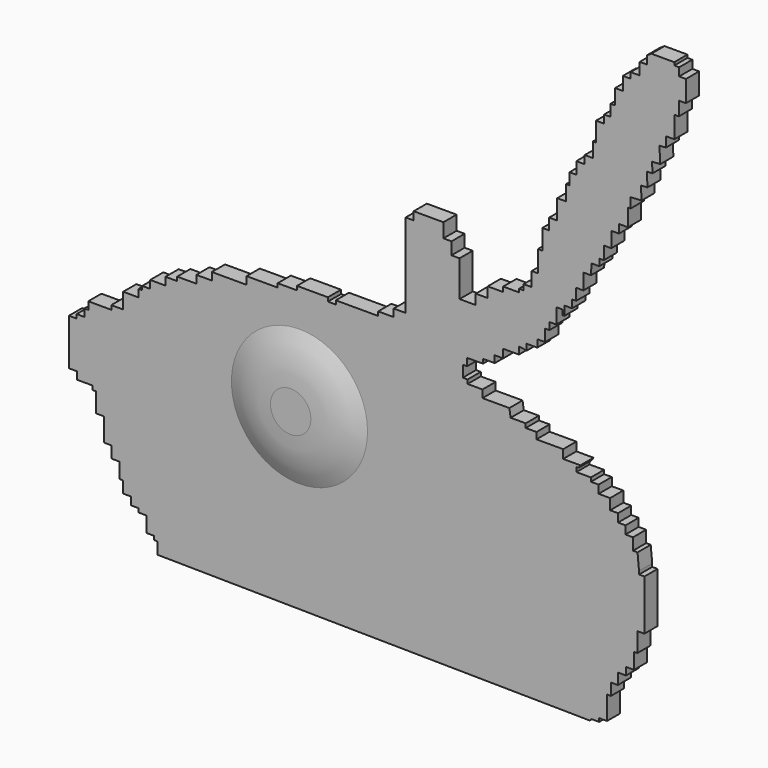
from build123d import *

# Parameters (mm, degrees)
F1_DEPTH = 0.762
F2_R     = 3.1487377101
F3_DEPTH = 0.508


# Not quite as in the source:
# - a fillet or chamfer that OpenCascade refuses, or shapes differently, is made with other operations: its cross-section is extruded or revolved along the edge and cut away or added


with BuildPart() as f1:
    # F0 (on Front) → F1 (new body)
    with BuildSketch(Plane.XZ):
        Polygon((-10.7027310878, 16.9802121818), (-10.7027310878, 16.4352189749), (9.2740571126, 16.1886904389), (9.361166507, 16.2728279829), (9.7121512517, 16.2728279829), (9.7121512517, 16.4274536073), (10.076017119, 16.4274536073), (10.076017119, 17.509419471), (10.2598499507, 17.509419471), (10.2598499507, 18.0550143123), (10.5776172131, 18.0550143123), (10.5776172131, 18.5661129653), (10.9531022608, 18.5661129653), (10.9531022608, 18.9169067889), (11.3242575899, 18.9169067889), (11.3242575899, 19.6492467076), (11.4805521443, 19.6492467076), (11.4805521443, 20.5453597009), (11.8060437962, 20.5453597009), (11.8060437962, 22.8735357523), (11.5571394563, 22.8735357523), (11.5571394563, 23.019047454), (11.4864483476, 23.7509682775), (11.2769883126, 23.7509682775), (11.2769883126, 24.2973826826), (10.9309256077, 24.2973826826), (10.9309256077, 24.6707666665), (10.5848629028, 24.6707666665), (10.5848629028, 25.0532571226), (10.2192526683, 25.0532571226), (10.2192526683, 25.5498923361), (9.6870232373, 25.5498923361), (9.6870232373, 25.9251333773), (9.330926463, 25.9251333773), (9.330926463, 26.1014979333), (8.6600910872, 26.1014979333), (8.6600910872, 26.3056345284), (8.7596448138, 26.3056345284), (8.8438820094, 26.4358203858), (8.0474531278, 26.4358203858), (8.0474531278, 26.8340352923), (6.8145194091, 26.8340352923), (6.8145194091, 27.1326974034), (6.3167512417, 27.1326974034), (6.3167512417, 27.3241456598), (5.6198756211, 27.3241456598), (5.5586118251, 27.699386701), (4.3180198409, 27.699386701), (4.3180198409, 28.0516538769), (3.6288024858, 28.0516538769), (3.6288024858, 28.2354447991), (3.4067214001, 28.2354447991), (3.4067214001, 28.7638437003), (3.6058286205, 28.7638437003), (3.6058286205, 29.108453542), (4.3409941718, 29.108453542), (4.3409941718, 29.3075609952), (4.8847105354, 29.3075609952), (4.8847105354, 29.6291969717), (5.2762227133, 29.6291969717), (5.2762227133, 30.0197526813), (6.0027744621, 30.0197526813), (6.0027744621, 30.3567033261), (6.3626994379, 30.2954409271), (6.3626994379, 30.5787846446), (6.8528093398, 30.5787846446), (6.8528093398, 30.9233944863), (7.2127343155, 30.9233944863), (7.2127343155, 31.4747691154), (7.4139898643, 31.4747691154), (7.4139898643, 31.8043418229), (7.7288472094, 31.8043418229), (7.7288472094, 32.5135849416), (8.0249523744, 32.5135849416), (8.0249523744, 32.2783663869), (8.1042656675, 32.2783663869), (8.1042656675, 32.7028520405), (8.4611764178, 32.7028520405), (8.4611764178, 33.0685973167), (8.6515294388, 33.0685973167), (8.6515294388, 33.5998237133), (8.9846476912, 33.5998237133), (8.9846476912, 34.3319140375), (9.3336272985, 34.3319140375), (9.3600647524, 34.8261408508), (9.7196195275, 34.8261408508), (9.7196195275, 35.1380035281), (9.9258357659, 35.1380035281), (9.9258357659, 35.7379503548), (10.2721722797, 35.7379503548), (10.2721722797, 36.4488959312), (10.6290839612, 36.4488959312), (10.6290839612, 36.8426926434), (11.0468016937, 36.8426926434), (11.0468016937, 37.5430695713), (11.0468016937, 37.6461409032), (11.1684938893, 37.6461409032), (11.1684938893, 38.1089963577), (11.6737550625, 38.1342493479), (11.6433482944, 38.742627176), (11.9479903872, 38.75785321), (11.9162704796, 39.3925043009), (12.1807143848, 39.4057212265), (12.1571606054, 39.8769846334), (12.5368040454, 39.8959592401), (12.4995354563, 40.6416282058), (12.7986464649, 40.6565777957), (12.7986464649, 41.1200486124), (13.1874894723, 41.1200486124), (13.1874894723, 42.1217381954), (13.3968675509, 42.1217381954), (13.3968675509, 42.7646152675), (13.7258889154, 42.7646152675), (13.7258889154, 43.7513552606), (13.4118227288, 43.7513552606), (13.4118227288, 44.1251210868), (13.1874894723, 44.1251210868), (13.1874894723, 44.2596748471), (12.1256476268, 44.2596748471), (11.9162704796, 44.1251210868), (11.9162704796, 43.7513552606), (11.5872481838, 43.7513552606), (11.5872481838, 43.1981831789), (11.1684938893, 43.1981831789), (11.1684938893, 42.929071933), (10.8095612377, 42.929071933), (10.8095612377, 42.3160977662), (10.4506285861, 42.3160977662), (10.4506285861, 41.6134186089), (10.2412505075, 41.6134186089), (10.2412505075, 41.0751961172), (9.9421404302, 41.0751961172), (9.9421404302, 40.7014340162), (9.567049332, 40.7014340162), (9.567049332, 39.8043952882), (9.4175431877, 39.8043952882), (9.4175431877, 39.1316190362), (9.0437782928, 39.1316190362), (9.0437782928, 38.75785321), (8.6550619453, 38.75785321), (8.6550619453, 38.2046811283), (8.3410982043, 38.2046811283), (8.3410982043, 37.6664586365), (8.1766415387, 37.6664586365), (8.1766415387, 36.9637794793), (7.7729751356, 36.9637794793), (7.7729751356, 36.0517911613), (7.399209775, 36.0517911613), (7.399209775, 35.5285182595), (7.0852469653, 35.5285182595), (7.0852469653, 34.6015803516), (6.8759382702, 34.6015803516), (6.8759382702, 33.6148403585), (6.5918765031, 33.6148403585), (6.5918765031, 32.9570136964), (6.2181116082, 32.9570136964), (6.2181116082, 32.7028520405), (6.0088024475, 32.7028520405), (6.0088024475, 32.553344965), (5.2762227133, 32.553344965), (5.2762227133, 32.3290862143), (4.5585935004, 32.3290862143), (4.5585935004, 31.8506658077), (4.0054204874, 31.8506658077), (4.0054204874, 31.3871987164), (3.2578899991, 31.3871987164), (3.2578899991, 33.0467149615), (2.8841246385, 33.0467149615), (2.8841246385, 33.6148403585), (2.5103592779, 33.6148403585), (2.5103592779, 34.2726670206), (1.1349029373, 34.2726670206), (1.1349029373, 33.8989011943), (0.7648753817, 33.8989011943), (0.7648753817, 30.0117395818), (0.2128840133, 30.0117395818), (0.2128840133, 29.662868008), (-0.5045263097, 29.662868008), (-0.5045263097, 29.4756293297), (-2.4671009742, 29.4756293297), (-2.4671009742, 29.3034724891), (-2.8314732481, 29.3034724891), (-2.8314732481, 29.4800959527), (-4.260267131, 29.4800959527), (-4.260267131, 29.2979851365), (-5.1528010517, 29.2979851365), (-5.1528010517, 29.1180480272), (-6.5885153599, 29.1180480272), (-6.5885153599, 28.7643931806), (-8.1972610205, 28.7643931806), (-8.1972610205, 28.415735811), (-8.9150499552, 28.415735811), (-8.9150499552, 28.0552376062), (-9.7993966192, 28.0552376062), (-9.7993966192, 27.8717204928), (-10.3413742036, 27.8717204928), (-10.3413742036, 27.5138057768), (-11.0485879704, 27.5138057768), (-11.0485879704, 27.1503776312), (-11.4187179133, 27.1503776312), (-11.4187179133, 26.9733015448), (-11.5851024166, 26.9733015448), (-11.5851024166, 26.627080515), (-12.2981043532, 26.627080515), (-12.2981043532, 25.904243812), (-12.8476871178, 25.904243812), (-12.8476871178, 25.7139522582), (-13.9118125662, 25.7139522582), (-13.9118125662, 25.3637637943), (-14.0915913507, 25.3637637943), (-14.0915913507, 25.0175409019), (-14.4485030323, 25.0175409019), (-14.4485030323, 24.8338580132), (-14.8080587387, 24.8338580132), (-14.8080587387, 22.6944163442), (-14.4432177767, 22.6944163442), (-14.4432177767, 22.3495159298), (-13.7267503887, 22.3495159298), (-13.7267503887, 22.1658330411), (-13.5496165603, 22.1658330411), (-13.5496165603, 21.265918389), (-13.1914103404, 21.265918389), (-13.1914103404, 20.1955363154), (-12.8319738433, 20.1955363154), (-12.8319738433, 19.6577031165), (-12.4698942527, 19.6577031165), (-12.4698942527, 18.9454331994), (-12.2981043532, 18.9454331994), (-12.2981043532, 18.4089224786), (-11.9370780885, 18.4089224786), (-11.9370780885, 18.0474910885), (-11.5851024166, 18.0474910885), (-11.5851024166, 17.869072035), (-11.2152853981, 17.869072035), (-11.2152853981, 17.1553902328), (-10.8714196831, 17.1553902328), (-10.8714196831, 16.9802121818), align=None)
    extrude(amount=-F1_DEPTH)

    # F2 (on face) → F3 (join)
    with BuildSketch(Plane.XZ):
        with Locations((-4.1458839551, 24.6049370617)):
            Circle(F2_R)
    extrude(amount=F3_DEPTH)

    # F4: fillet of radius 5.08 on 1 edges, made by hand

    # F4_s1 → F4_t2 (revolve, cut)
    with BuildSketch(Plane.XY.offset(24.6049370617)):
        with BuildLine():
            ThreePointArc((-0.9971462449, 0), (-2.0755443757, -0.3793715272), (-3.2114669082, -0.508))
            Line((-3.2114669082, -0.508), (-3.2114669082, -0.6096))
            Line((-3.2114669082, -0.6096), (-0.9971462449, -0.6096))
            Line((-0.9971462449, -0.6096), (-0.8955462449, -0.508))
            ThreePointArc((-0.8955462449, -0.508), (-0.8955462449, -0.254), (-0.9528598317, -0.09144))
            Line((-0.9528598317, -0.09144), (-0.9971462449, 0))
        make_face()
    revolve(axis=Axis((-4.1458839551, -0.508, 24.6049370617), (0, -1, 0)), mode=Mode.SUBTRACT)


solid = f1.part
